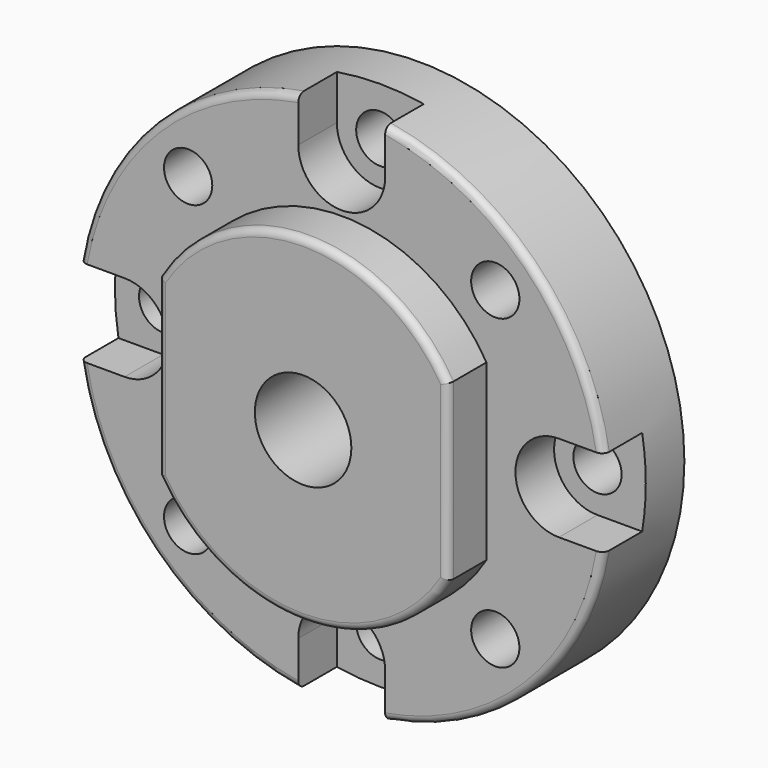
from build123d import *

# Parameters (mm, degrees)
F0_R      = 11
F1_DEPTH  = 6
F2_R      = 16
F3_DEPTH  = 2
F5_R      = 1
F6_DEPTH  = 4.001
F9_DEPTH  = 2
F10_R     = 0.3
F11_R     = 6.15
F12_DEPTH = 1
F4_R      = 2
F13_DEPTH = 7.001


with BuildPart() as f1:
    # F0 (on Front) → F1 (new body)
    with BuildSketch(Plane.XZ):
        Circle(F0_R)
    extrude(amount=F1_DEPTH)

    # F2 (on face) → F3 (cut)
    with BuildSketch(Plane.XZ.offset(6)):
        Circle(F2_R)
        with BuildLine():
            ThreePointArc((6, -3.6055512755), (0, -7), (-6, -3.6055512755))
            Line((-6, -3.6055512755), (-6, 3.6055512755))
            ThreePointArc((-6, 3.6055512755), (0, 7), (6, 3.6055512755))
            Line((6, 3.6055512755), (6, -3.6055512755))
        make_face(mode=Mode.SUBTRACT)
    extrude(amount=-F3_DEPTH, mode=Mode.SUBTRACT)

    # F5 (on face) → F6 (cut, through all)
    with BuildSketch(Plane.XZ.offset(4)):
        with Locations((0, 9)):
            Circle(F5_R)
        with Locations((-6.3639610307, 6.3639610307)):
            Circle(F5_R)
        with Locations((-9, 0)):
            Circle(F5_R)
        with Locations((-6.3639610307, -6.3639610307)):
            Circle(F5_R)
        with Locations((0, -9)):
            Circle(F5_R)
        with Locations((6.3639610307, -6.3639610307)):
            Circle(F5_R)
        with Locations((9, 0)):
            Circle(F5_R)
        with Locations((6.3639610307, 6.3639610307)):
            Circle(F5_R)
    extrude(amount=-F6_DEPTH, mode=Mode.SUBTRACT)

    # F8 (on face) → F9 (cut)
    with BuildSketch(Plane.XZ.offset(4)):
        with BuildLine():
            Line((-1.8, 11.6544359102), (-1.8, 9))
            ThreePointArc((-1.8, 9), (0, 7.2), (1.8, 9))
            Line((1.8, 9), (1.8, 11.6544359102))
            Line((1.8, 11.6544359102), (-1.8, 11.6544359102))
        make_face()
        with BuildLine():
            Line((-11.6544359102, -1.8), (-9, -1.8))
            ThreePointArc((-9, -1.8), (-7.2, 0), (-9, 1.8))
            Line((-9, 1.8), (-11.6544359102, 1.8))
            Line((-11.6544359102, 1.8), (-11.6544359102, -1.8))
        make_face()
        with BuildLine():
            Line((1.8, -11.6544359102), (1.8, -9))
            ThreePointArc((1.8, -9), (0, -7.2), (-1.8, -9))
            Line((-1.8, -9), (-1.8, -11.6544359102))
            Line((-1.8, -11.6544359102), (1.8, -11.6544359102))
        make_face()
        with BuildLine():
            Line((11.6544359102, 1.8), (9, 1.8))
            ThreePointArc((9, 1.8), (7.2, 0), (9, -1.8))
            Line((9, -1.8), (11.6544359102, -1.8))
            Line((11.6544359102, -1.8), (11.6544359102, 1.8))
        make_face()
    extrude(amount=-F9_DEPTH, mode=Mode.SUBTRACT)

    # F10
    f10_edges = [f1.edges().sort_by_distance(p)[0] for p in [
        (0, -6, -7),
        (-6, -6, 0),
        (6, -6, 0),
        (0, -6, 7),
        (7.778175, -4, -7.778175),
        (-7.778175, -4, -7.778175),
        (-7.778175, -4, 7.778175),
        (7.778175, -4, 7.778175),
    ]]
    fillet(f10_edges, radius=F10_R)

    # F11 (on face) → F12 (join)
    with BuildSketch(Plane(origin=(0, 0, 0), x_dir=(-1, 0, 0), z_dir=(0, 1, 0))):
        Circle(F11_R)
    extrude(amount=F12_DEPTH)

    # F4 (on face) → F13 (cut, through all)
    with BuildSketch(Plane.XZ.offset(6)):
        Circle(F4_R)
    extrude(amount=-F13_DEPTH, mode=Mode.SUBTRACT)


solid = f1.part
